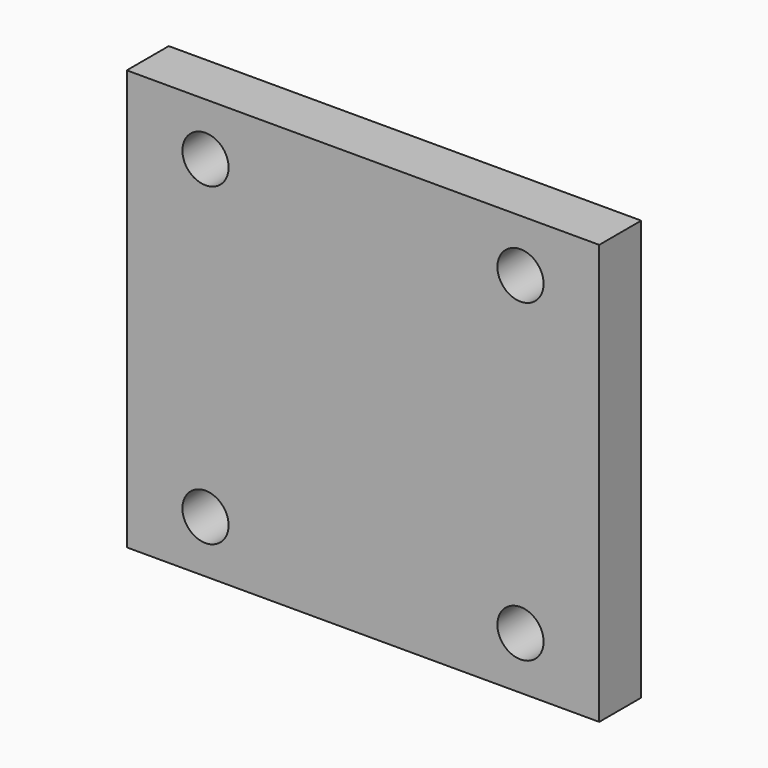
from build123d import *

# Parameters (mm, degrees)
F0_W     = 28.575
F0_H     = 25.4
F1_DEPTH = 3.175
F3_D     = 2.794


# Not quite as in the source:
# - a length typed as a fraction of an inch, garbled in the dataset ("3 / 203.2 mm" for 3/8 in), is restored


with BuildPart() as f1:
    # F0 (on Front) → F1 (new body)
    with BuildSketch(Plane.XZ):
        Rectangle(F0_W, F0_H)
    extrude(amount=F1_DEPTH)

    # F3 (through all)
    with Locations(Plane(origin=(0, 0, 0), x_dir=(-1, 0, 0), z_dir=(0, 1, 0))):
        with Locations((9.525, -9.525), (-9.525, -9.525), (-9.525, 9.525), (9.525, 9.525)):
            Hole(F3_D / 2)


solid = f1.part
